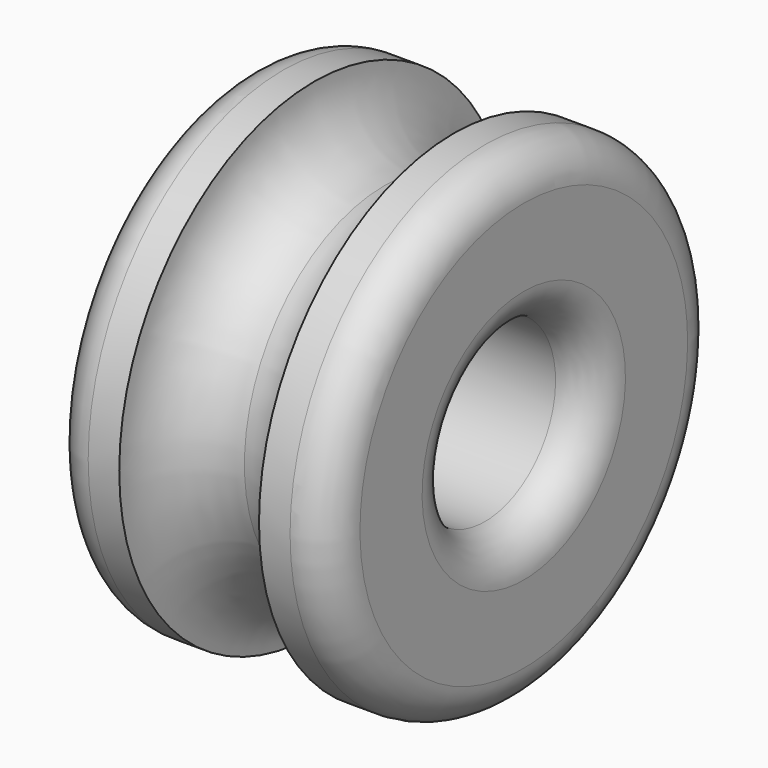
from build123d import *
from build123d import SkipClean  # not in build123d's __all__


# Not quite as in the source:
# - a feature of the source that left no trace in its solid (it failed there, or was rolled back) is left out
# - the program builds the solid bodies; features that only make, move or delete a surface that nothing else refers to are left out


with BuildPart() as f3:
    # F2 (on Front) → F3 (revolve)
    with BuildSketch(Plane.XZ):
        with BuildLine():
            ThreePointArc((8.9994186326, 31.3704956104), (6.3276909161, 25.0727650489), (0, 22.4727906481))
            Line((0, 22.4727906481), (0, 11.3704956104))
            Line((0, 11.3704956104), (12.9994186326, 11.3704956104))
            ThreePointArc((12.9994186326, 11.3704956104), (16.5349525386, 12.8349617044), (17.9994186326, 16.3704956104))
            Line((17.9994186326, 16.3704956104), (17.9994186326, 26.3704956104))
            ThreePointArc((17.9994186326, 26.3704956104), (16.5349525386, 29.9060295163), (12.9994186326, 31.3704956104))
            Line((12.9994186326, 31.3704956104), (8.9994186326, 31.3704956104))
        make_face()
    revolve(axis=Axis((1.0410054399, 0, 0), (-1, 0, 0)))

    # F0: F3 across plane


with BuildPart() as f3_1:
    add(f3.part, clean=False)
    with SkipClean():  # cleaning this boolean's faces spoils the solid; the shape is the same uncleaned
        add(f3.part.mirror(Plane.YZ), clean=False)


solid = f3_1.part
